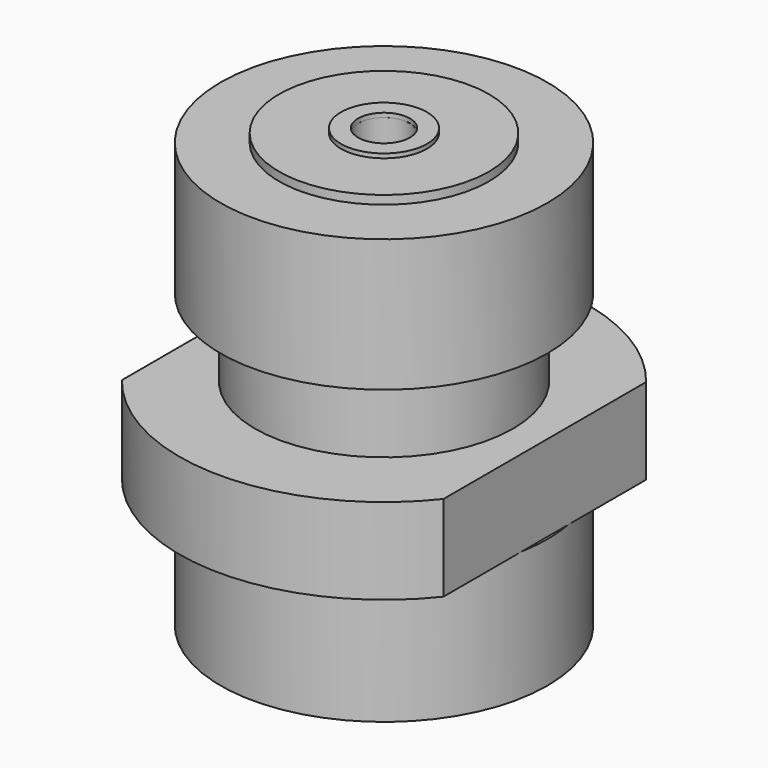
from build123d import *

# Parameters (mm, degrees)
F1_DEPTH  = 1.27
F2_R      = 2.413
F3_DEPTH  = 1.905
F4_R      = 1.905
F5_DEPTH  = 1.143
F6_R      = 2.413
F7_DEPTH  = 1.9558
F8_R      = 1.5494
F9_DEPTH  = 6.5532
F11_R     = 0.635
F12_DEPTH = 6.6548
F14_R     = 0.3825855741
F15_DEPTH = 1.27
F16_R     = 0.38227
F17_DEPTH = 1.27
F18_R     = 0.38227
F19_DEPTH = 1.27


with BuildPart() as f1:
    # F0 (on Top) → F1 (new body)
    with BuildSketch(Plane.XY):
        with BuildLine():
            Line((2.3749, -1.8697488468), (2.3749, 1.8697488468))
            ThreePointArc((2.3749, 1.8697488468), (0, 3.0226), (-2.3749, 1.8697488468))
            Line((-2.3749, 1.8697488468), (-2.3749, -1.8697488468))
            ThreePointArc((-2.3749, -1.8697488468), (0, -3.0226), (2.3749, -1.8697488468))
        make_face()
    extrude(amount=F1_DEPTH)

    # F2 (on face) → F3 (join)
    with BuildSketch(Plane(origin=(0, 0, 0), x_dir=(1, 0, 0), z_dir=(0, 0, -1))):
        Circle(F2_R)
    extrude(amount=F3_DEPTH)

    # F4 (on face) → F5 (join)
    with BuildSketch(Plane.XY.offset(1.27)):
        Circle(F4_R)
    extrude(amount=F5_DEPTH)

    # F6 (on face) → F7 (join)
    with BuildSketch(Plane.XY.offset(2.413)):
        Circle(F6_R)
    extrude(amount=F7_DEPTH)

    # F18 (on face) → F19 (cut)
    with BuildSketch(Plane.XY.offset(4.3688)):
        Circle(F18_R)
    extrude(amount=-F19_DEPTH, mode=Mode.SUBTRACT)


with BuildPart() as f9:
    # F8 (on face) → F9 (new body)
    with BuildSketch(Plane.XY.offset(4.3688)):
        Circle(F8_R)
    extrude(amount=-F9_DEPTH)


with BuildPart() as f9_1:
    # F10: moved
    add(f9.part.moved(Location((0, 0, 0.127))))

    # F16 (on face) → F17 (cut)
    with BuildSketch(Plane.XY.offset(4.4958)):
        Circle(F16_R)
    extrude(amount=-F17_DEPTH, mode=Mode.SUBTRACT)


with BuildPart() as f12:
    # F11 (on face) → F12 (new body)
    with BuildSketch(Plane.XY.offset(4.4958)):
        Circle(F11_R)
    extrude(amount=-F12_DEPTH)


with BuildPart() as f12_1:
    # F13: moved
    add(f12.part.moved(Location((0, 0, 0.0635))))

    # F14 (on face) → F15 (cut)
    with BuildSketch(Plane.XY.offset(4.5593)):
        Circle(F14_R)
    extrude(amount=-F15_DEPTH, mode=Mode.SUBTRACT)


solid = Compound([f1.part, f9_1.part, f12_1.part])
